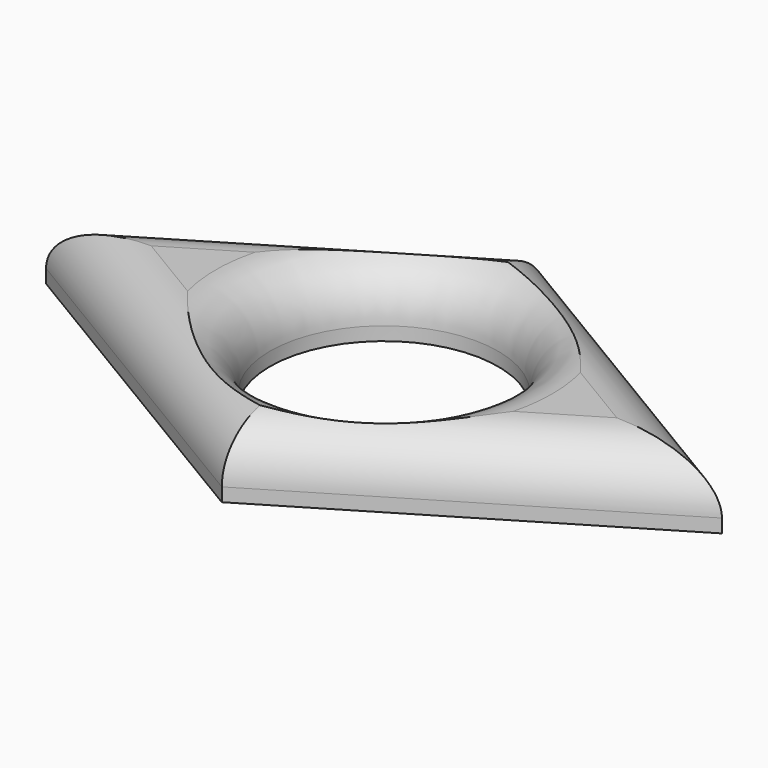
from build123d import *

# Parameters (mm, degrees)
F2_DEPTH     = 25.4
F3_DEPTH     = 19.05
F4_D         = 21.4376
F5_T1_DEPTH  = 62.4265445323
F5_T3_DEPTH  = 62.4265445323
F5_T5_DEPTH  = 62.4265445323
F5_T7_DEPTH  = 62.4265445323
F6_TEXT_SIZE = 4.3528232103
F7_DEPTH     = 1.27


# Not quite as in the source:
# - a fillet or chamfer that OpenCascade refuses, or shapes differently, is made with other operations: its cross-section is extruded or revolved along the edge and cut away or added
# - Text() gives the source's letters only with a copy of the font that has no kerning and outlines rounded to 1/6400 em; it was checked with that copy


with BuildPart() as f2:
    # F1 (on face) → F2 (new body)
    with BuildSketch(Plane.XY):
        Polygon((31.75, 19.05), (31.75, 38.1), (0, 19.05), align=None)
        Polygon((63.5, 19.05), (31.75, 38.1), (31.75, 19.05), align=None)
        Polygon((31.75, 19.05), (0, 19.05), (31.75, 0), align=None)
        Polygon((63.5, 19.05), (31.75, 19.05), (31.75, 0), align=None)
    extrude(amount=F2_DEPTH)

    # F3 (cut): a face of the model
    f3_faces = [f2.faces().sort_by_distance(p)[0] for p in [
        (31.75, 19.05, 25.4),
    ]]
    extrude(f3_faces, amount=-F3_DEPTH, mode=Mode.SUBTRACT)

    # F4 (through all)
    with Locations(Plane(origin=(0, 0, 0), x_dir=(1, 0, 0), z_dir=(0, 0, -1))):
        with Locations((31.75, -19.05)):
            Hole(F4_D / 2)

    # F5: fillet of radius 5.08 on 5 edges, made by hand

    # F5_s2 → F5_t1 (cut)
    with BuildSketch(Plane(origin=(51.0445719213, 30.6267431528, 0), x_dir=(0, 0, 1), z_dir=(-0.8574929257, -0.5144957554, 0))):
        with BuildLine():
            ThreePointArc((1.27, 16.3352402348), (4.8621024484, 14.8473426833), (6.35, 11.2552402348))
            Line((6.35, 11.2552402348), (6.35, 16.3352402348))
            Line((6.35, 16.3352402348), (1.27, 16.3352402348))
        make_face()
    extrude(amount=F5_T1_DEPTH, mode=Mode.SUBTRACT)

    # F5_s4 → F5_t3 (cut)
    with BuildSketch(Plane(origin=(49.1769248624, -29.5061549175, 0), x_dir=(0, 0, 1), z_dir=(-0.8574929257, 0.5144957554, 0))):
        with BuildLine():
            ThreePointArc((6.35, 43.9257207045), (4.8621024484, 47.5178231529), (1.27, 49.0057207045))
            Line((1.27, 49.0057207045), (6.35, 49.0057207045))
            Line((6.35, 49.0057207045), (6.35, 43.9257207045))
        make_face()
    extrude(amount=F5_T3_DEPTH, mode=Mode.SUBTRACT)

    # F5_s6 → F5_t5 (cut)
    with BuildSketch(Plane(origin=(-19.2945719213, 11.5767431528, 0), x_dir=(0, 0, 1), z_dir=(0.8574929257, -0.5144957554, 0))):
        with BuildLine():
            ThreePointArc((1.27, -16.3352402348), (4.8621024484, -17.8231377864), (6.35, -21.4152402348))
            Line((6.35, -21.4152402348), (6.35, -16.3352402348))
            Line((6.35, -16.3352402348), (1.27, -16.3352402348))
        make_face()
    extrude(amount=F5_T5_DEPTH, mode=Mode.SUBTRACT)

    # F5_s8 → F5_t7 (cut)
    with BuildSketch(Plane(origin=(12.4554280787, 7.4732568472, 0), x_dir=(0, 0, 1), z_dir=(0.8574929257, 0.5144957554, 0))):
        with BuildLine():
            ThreePointArc((6.35, 11.2552402348), (4.8621024484, 14.8473426833), (1.27, 16.3352402348))
            Line((1.27, 16.3352402348), (6.35, 16.3352402348))
            Line((6.35, 16.3352402348), (6.35, 11.2552402348))
        make_face()
    extrude(amount=F5_T7_DEPTH, mode=Mode.SUBTRACT)

    # F5_s9 → F5_t10 (revolve, cut)
    with BuildSketch(Plane.XZ.offset(-19.05)):
        with BuildLine():
            ThreePointArc((47.5488, 6.35), (43.9566975516, 4.8621024484), (42.4688, 1.27))
            Line((42.4688, 1.27), (42.4688, 6.35))
            Line((42.4688, 6.35), (47.5488, 6.35))
        make_face()
    revolve(axis=Axis((31.75, 19.05, 6.35), (0, 0, -1)), mode=Mode.SUBTRACT)

    # F6 (on face) → F7 (join)
    with BuildSketch(Plane(origin=(0, 0, 0), x_dir=(1, 0, 0), z_dir=(0, 0, -1))):
        with Locations((7.374192588, -20.4633884132)):
            Text('R.S', F6_TEXT_SIZE, font='Open Sans', text_align=(TextAlign.LEFT, TextAlign.BOTTOM))
    extrude(amount=F7_DEPTH)


solid = f2.part
